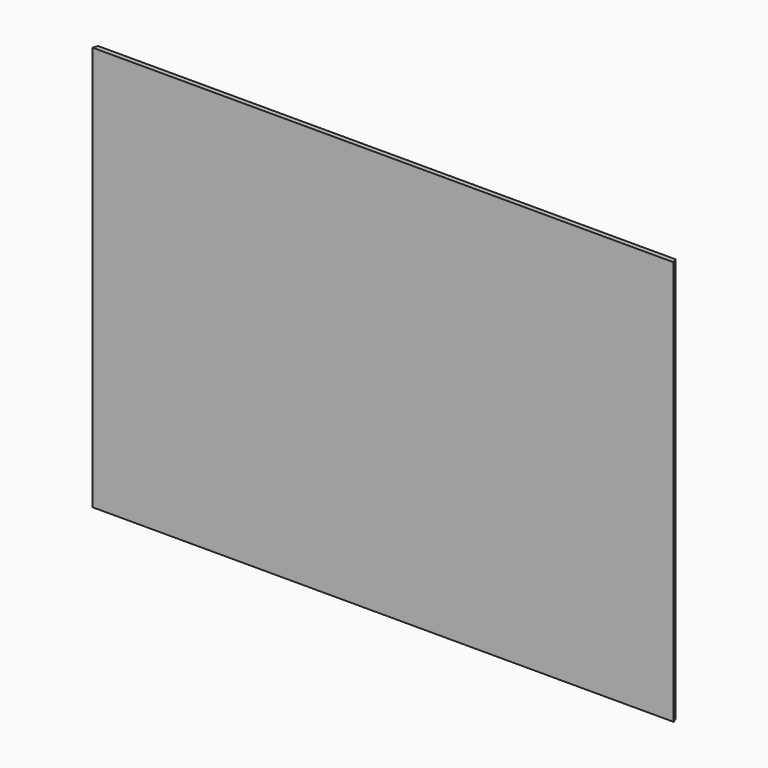
from build123d import *

# Parameters (mm, degrees)
F0_W       = 1514.0918044843
F0_H       = 1054.1
F1_DEPTH   = 12.7
F2_SIZE2   = 5.260502
F2_SIZE    = 12.69999
F2_2_SIZE2 = 5.260502
F2_2_SIZE  = 12.69999


# Not quite as in the source:
# - a fillet or chamfer is up to 0.001 mm smaller than in the source, because OpenCascade refuses the exact size


with BuildPart() as f1:
    # F0 (on Front) → F1 (new body)
    with BuildSketch(Plane.XZ):
        with Locations((757.0459022421, 527.05)):
            Rectangle(F0_W, F0_H)
    extrude(amount=-F1_DEPTH)

    # F2 (size 12.7 and 5.2605122421 in the source; OpenCascade refuses exactly that, so slightly less here)
    f2_edges = [f1.edges().sort_by_distance(p)[0] for p in [
        (1514.091804, 12.7, 527.05),
    ]]
    f2_side = f1.faces().sort_by_distance((1514.091804, 6.35, 527.05))[0]
    chamfer(f2_edges, length=F2_SIZE, length2=F2_SIZE2, reference=f2_side)

    # F2#2 (size 12.7 and 5.2605122421 in the source; OpenCascade refuses exactly that, so slightly less here)
    f2_2_edges = [f1.edges().sort_by_distance(p)[0] for p in [
        (0, 12.7, 527.05),
    ]]
    f2_2_side = f1.faces().sort_by_distance((0, 6.35, 527.05))[0]
    chamfer(f2_2_edges, length=F2_2_SIZE, length2=F2_2_SIZE2, reference=f2_2_side)


solid = f1.part
